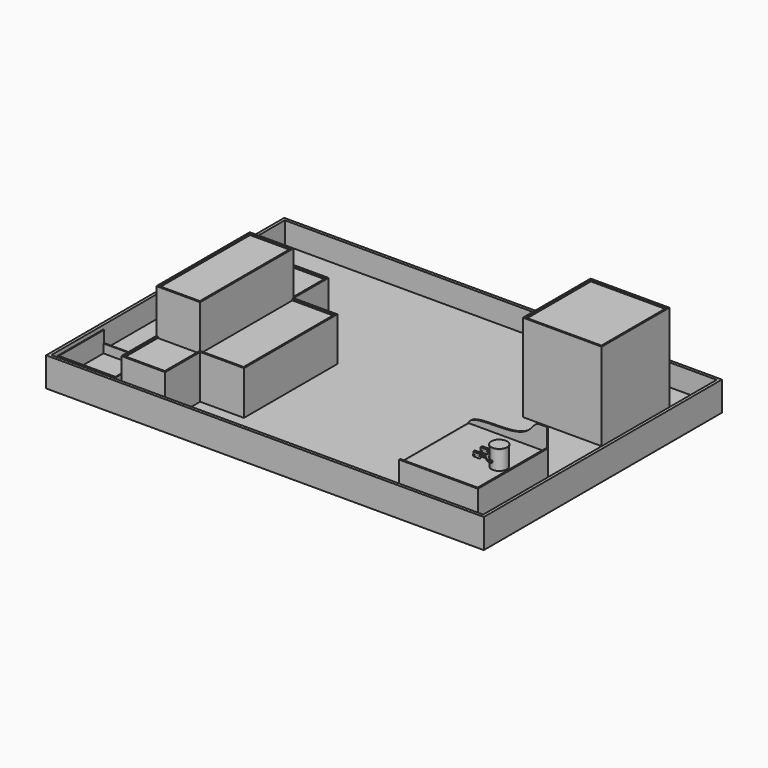
from build123d import *

# Parameters (mm, degrees)
F0_R       = 27.2
F1_DEPTH   = 2.83
F2_R       = 26.4
F3_DEPTH   = 67.36
F4_R       = 27.2
F5_DEPTH   = 2.83
F9_W       = 270
F9_H       = 300
F10_DEPTH  = 72
F12_DEPTH  = 15
F14_DEPTH  = 5
F15_W      = 5
F15_H      = 290
F16_DEPTH  = 5
F17_W      = 1500
F17_H      = 1020
F18_DEPTH  = 25
F19_W      = 270
F19_H      = 290
F20_DEPTH  = 300
F21_W      = 260
F21_H      = 280
F22_DEPTH  = 5
F23_W      = 1500
F23_H      = 1020
F23_W_2    = 1480
F23_H_2    = 1000
F24_DEPTH  = 75
F26_DEPTH  = 150
F27_W      = 150
F27_H      = 400
F28_DEPTH  = 150
F29_W      = 140
F29_H      = 390
F30_DEPTH  = 5
F31_W      = 140
F31_H      = 145
F31_W_2    = 145
F31_H_2    = 390
F32_DEPTH  = 5
F33_R      = 3
F34_DEPTH  = 4
F35_R      = 3.99999
F35_2_R    = 3.99999
F36_R      = 3
F37_DEPTH  = 8
F38_R      = 3
F39_DEPTH  = 8
F40_R      = 3
F40_R_2    = 2.5
F41_DEPTH  = 3
F42_R      = 3
F42_R_2    = 2.5
F43_DEPTH  = 3
F45_DEPTH  = 270.001
F46_W      = 200
F46_H      = 200
F46_W_2    = 194
F46_H_2    = 191
F47_DEPTH  = 30
F49_DEPTH  = 40
F50_R      = 3.0302739223
F50_R_2    = 2.9857883715
F50_R_3    = 3.0752405993
F50_R_4    = 2.9957966751
F10_FACE_W = 260
F10_FACE_H = 290
F51_DEPTH  = 6


# Not quite as in the source:
# - a fillet or chamfer is up to 0.001 mm smaller than in the source, because OpenCascade refuses the exact size
# - a feature names something its author has since deleted; it is built from what else it names


with BuildPart() as f1:
    # F0 (on Top) → F1 (new body)
    with BuildSketch(Plane.XY):
        Circle(F0_R)
    extrude(amount=F1_DEPTH)

    # F2 (on face) → F3 (join)
    with BuildSketch(Plane.XY.offset(2.83)):
        Circle(F2_R)
    extrude(amount=F3_DEPTH)

    # F4 (on face) → F5 (join)
    with BuildSketch(Plane.XY.offset(70.19)):
        Circle(F4_R)
    extrude(amount=F5_DEPTH)


with BuildPart() as f10:
    # F9 (on Top) → F10 (new body)
    with BuildSketch(Plane.XY):
        with Locations((-87.8, 0)):
            Rectangle(F9_W, F9_H)
    extrude(amount=-F10_DEPTH)

    # F11 (on face) → F12 (join)
    with BuildSketch(Plane.XY):
        Polygon((-222.8, -145), (-222.8, -150), (47.2, -150), (47.2, 150), (42.2, 150), (42.2, -145), align=None)
    extrude(amount=F12_DEPTH)

    # F13 (on face) → F14 (join)
    with BuildSketch(Plane(origin=(0, 150, 0), x_dir=(-1, 0, 0), z_dir=(0, 1, 0))):
        with BuildLine():
            Line((-21.3134280931, 81.3575685024), (-47.2, 81.3575685024))
            Line((-47.2, 81.3575685024), (-47.2, -72))
            Line((-47.2, -72), (222.8, -72))
            Line((222.8, -72), (222.8, 0))
            add(Edge.make_bspline(
                [(-21.3134280931, 81.3575685024), (-6.3059147253, 81.3822787863), (12.9585432644, 38.1268753575), (103.6097013063, 23.6068887567), (223.0224295336, 30.7718731823), (222.8, 0)],
                knots=[0, 0, 0, 0, 0.2487100673, 0.6151112321, 1, 1, 1, 1], degree=3))
        make_face()
    extrude(amount=-F14_DEPTH)

    # F15 (on face) → F16 (join)
    with BuildSketch(Plane.XY):
        with Locations((-220.3, 0)):
            Rectangle(F15_W, F15_H)
    extrude(amount=F16_DEPTH)

    # F17 (on face) → F18 (join)
    with BuildSketch(Plane(origin=(0, 0, -72), x_dir=(1, 0, 0), z_dir=(0, 0, -1))):
        with Locations((-602.8, -260)):
            Rectangle(F17_W, F17_H)
    extrude(amount=F18_DEPTH)

    # F19 (on face) → F20 (join)
    with BuildSketch(Plane.XY.offset(-72)):
        with Locations((-87.8, 525)):
            Rectangle(F19_W, F19_H)
    extrude(amount=F20_DEPTH)

    # F21 (on face) → F22 (cut)
    with BuildSketch(Plane.XY.offset(228)):
        with Locations((-87.8, 525)):
            Rectangle(F21_W, F21_H)
    extrude(amount=-F22_DEPTH, mode=Mode.SUBTRACT)

    # F23 (on face) → F24 (join)
    with BuildSketch(Plane.XY.offset(-72)):
        with Locations((-602.8, 260)):
            Rectangle(F23_W, F23_H)
        with Locations((-602.8, 260)):
            Rectangle(F23_W_2, F23_H_2, mode=Mode.SUBTRACT)
    extrude(amount=F24_DEPTH)

    # F25 (on face) → F26 (join)
    with BuildSketch(Plane.XY.offset(-72)):
        Polygon((-952.8, 460), (-1102.8, 460), (-1102.8, -240), (-952.8, -240), (-952.8, -90), (-802.8, -90), (-802.8, 310), (-952.8, 310), align=None)
    extrude(amount=F26_DEPTH)

    # F27 (on face) → F28 (join)
    with BuildSketch(Plane.XY.offset(78)):
        with Locations((-1027.8, 110)):
            Rectangle(F27_W, F27_H)
    extrude(amount=F28_DEPTH)

    # F29 (on face) → F30 (cut)
    with BuildSketch(Plane.XY.offset(228)):
        with Locations((-1027.8, 110)):
            Rectangle(F29_W, F29_H)
    extrude(amount=-F30_DEPTH, mode=Mode.SUBTRACT)

    # F31 (on face) → F32 (cut)
    with BuildSketch(Plane.XY.offset(78)):
        with Locations((-1027.8, 382.5)):
            Rectangle(F31_W, F31_H)
        with Locations((-880.3, 110)):
            Rectangle(F31_W_2, F31_H_2)
        with Locations((-1027.8, -162.5)):
            Rectangle(F31_W, F31_H)
    extrude(amount=-F32_DEPTH, mode=Mode.SUBTRACT)

    # F46 (on face) → F47 (join)
    with BuildSketch(Plane.XY.offset(-72)):
        with Locations((-1232.8, -130)):
            Rectangle(F46_W, F46_H)
        with Locations((-1232.8, -128.5)):
            Rectangle(F46_W_2, F46_H_2, mode=Mode.SUBTRACT)
    extrude(amount=F47_DEPTH)

    # F48 (on face) → F49 (join)
    with BuildSketch(Plane.XY.offset(-42)):
        Polygon((-1329.8, -30), (-1332.8, -30), (-1332.8, -230), (-1329.8, -230), (-1135.8, -230), (-1132.8, -230), (-1132.8, -30), (-1135.8, -30), (-1135.8, -224), (-1329.8, -224), align=None)
    extrude(amount=F49_DEPTH)


with BuildPart() as f34:
    # F33 (on offset) → F34 (new body, symmetric)
    with BuildSketch(Plane.XY.offset(25)):
        with BuildLine():
            Line((-55, -12), (-74.5, -12))
            Line((-74.5, -12), (-74.5, -13))
            Line((-74.5, -13), (-65.6457513111, -13))
            ThreePointArc((-65.6457513111, -13), (-67, -16), (-65.6457513111, -19))
            Line((-65.6457513111, -19), (-74.5, -19))
            Line((-74.5, -19), (-74.5, -20))
            Line((-74.5, -20), (-55, -20))
            ThreePointArc((-55, -20), (-51, -16), (-55, -12))
        make_face()
        with Locations((-63, -16)):
            Circle(F33_R, mode=Mode.SUBTRACT)
        with Locations((-55, -16)):
            Circle(F33_R, mode=Mode.SUBTRACT)
    extrude(amount=F34_DEPTH, both=True)

    # F35 (radius 4 in the source; OpenCascade refuses exactly that, so slightly less here)
    f35_edges = [f34.edges().sort_by_distance(p)[0] for p in [
        (-74.5, -19.5, 29),
        (-74.5, -12.5, 29),
        (-74.5, -19.5, 21),
        (-74.5, -12.5, 21),
    ]]
    fillet(f35_edges, radius=F35_R)

    # F36 (on face) → F37 (join, through all)
    with BuildSketch(Plane.XZ.offset(20)):
        with Locations((-70.5, 25)):
            Circle(F36_R)
    extrude(amount=-F37_DEPTH)

    # F42 (on offset) → F43 (join, symmetric)
    with BuildSketch(Plane.XY.offset(25)):
        with Locations((-63, -16)):
            Circle(F42_R)
        with Locations((-63, -16)):
            Circle(F42_R_2, mode=Mode.SUBTRACT)
        with Locations((-55, -16)):
            Circle(F42_R)
        with Locations((-55, -16)):
            Circle(F42_R_2, mode=Mode.SUBTRACT)
    extrude(amount=F43_DEPTH, both=True)


with BuildPart() as f34b:
    # F33 (on offset) → F34, piece 2 (new body, symmetric)
    with BuildSketch(Plane.XY.offset(25)):
        with BuildLine():
            Line((-74.5, 13), (-74.5, 12))
            Line((-74.5, 12), (-55, 12))
            ThreePointArc((-55, 12), (-51, 16), (-55, 20))
            Line((-55, 20), (-74.5, 20))
            Line((-74.5, 20), (-74.5, 19))
            Line((-74.5, 19), (-65.6457513111, 19))
            ThreePointArc((-65.6457513111, 19), (-67, 16), (-65.6457513111, 13))
            Line((-65.6457513111, 13), (-74.5, 13))
        make_face()
        with Locations((-63, 16)):
            Circle(F33_R, mode=Mode.SUBTRACT)
        with Locations((-55, 16)):
            Circle(F33_R, mode=Mode.SUBTRACT)
    extrude(amount=F34_DEPTH, both=True)

    # F35#2 (radius 4 in the source; OpenCascade refuses exactly that, so slightly less here)
    f35_2_edges = [f34b.edges().sort_by_distance(p)[0] for p in [
        (-74.5, 12.5, 29),
        (-74.5, 19.5, 29),
        (-74.5, 19.5, 21),
        (-74.5, 12.5, 21),
    ]]
    fillet(f35_2_edges, radius=F35_2_R)

    # F38 (on face) → F39 (join, through all)
    with BuildSketch(Plane(origin=(0, 20, 0), x_dir=(-1, 0, 0), z_dir=(0, 1, 0))):
        with Locations((70.5, 25)):
            Circle(F38_R)
    extrude(amount=-F39_DEPTH)

    # F40 (on offset) → F41 (join, symmetric)
    with BuildSketch(Plane.XY.offset(25)):
        with Locations((-55, 16)):
            Circle(F40_R)
        with Locations((-55, 16)):
            Circle(F40_R_2, mode=Mode.SUBTRACT)
        with Locations((-63, 16)):
            Circle(F40_R)
        with Locations((-63, 16)):
            Circle(F40_R_2, mode=Mode.SUBTRACT)
    extrude(amount=F41_DEPTH, both=True)


with BuildPart() as f45_tool:
    # F44 (on face) → F45 (new body, through all)
    with BuildSketch(Plane(origin=(0, 20, 0), x_dir=(-1, 0, 0), z_dir=(0, 1, 0))):
        with BuildLine():
            Line((71.5, 26), (71.5, 27.2912878475))
            ThreePointArc((71.5, 27.2912878475), (70.5, 27.5), (69.5, 27.2912878475))
            Line((69.5, 27.2912878475), (69.5, 26))
            Line((69.5, 26), (68.2087121525, 26))
            ThreePointArc((68.2087121525, 26), (68, 25), (68.2087121525, 24))
            Line((68.2087121525, 24), (69.5, 24))
            Line((69.5, 24), (69.5, 22.7087121525))
            ThreePointArc((69.5, 22.7087121525), (70.5, 22.5), (71.5, 22.7087121525))
            Line((71.5, 22.7087121525), (71.5, 24))
            Line((71.5, 24), (72.7912878475, 24))
            ThreePointArc((72.7912878475, 24), (73, 25), (72.7912878475, 26))
            Line((72.7912878475, 26), (71.5, 26))
        make_face()
    extrude(amount=-F45_DEPTH)


with BuildPart() as f34_1:
    add(f34.part)

    # F45: cut by f45_tool
    add(f45_tool.part, mode=Mode.SUBTRACT)


with BuildPart() as f34b_1:
    add(f34b.part)

    # F45: cut by f45_tool
    add(f45_tool.part, mode=Mode.SUBTRACT)


with BuildPart() as f51:
    # F50 (on face) + F10_face (on face) → F51 (new body)
    with BuildSketch(Plane.XY.offset(29)):
        with BuildLine():
            ThreePointArc((-71.9986608624, 19.9992600828), (-74.119981206, 19.1205804264), (-74.9986608624, 16.9992600828))
            Line((-74.9986608624, 16.9992600828), (-74.9986608624, 14.9319520891))
            ThreePointArc((-74.9986608624, 14.9319520891), (-74.119981206, 12.8106317455), (-71.9986608624, 11.9319520891))
            Line((-71.9986608624, 11.9319520891), (-33.2765181611, 11.9319520891))
            ThreePointArc((-33.2765181611, 11.9319520891), (-35.5474344403, -0.0287606514), (-33.3410842856, -12.0015518465))
            Line((-33.3410842856, -12.0015518465), (-71.5077546412, -12.0054899377))
            ThreePointArc((-71.5077546412, -12.0054899377), (-73.6288748781, -12.8842790214), (-74.507445097, -15.0054899217))
            Line((-74.507445097, -15.0054899217), (-74.507445097, -17.0043950344))
            ThreePointArc((-74.507445097, -17.0043950344), (-73.6286559973, -19.1258248155), (-71.5071355527, -20.0043950184))
            Line((-71.5071355527, -20.0043950184), (-28.9120785892, -20))
            ThreePointArc((-28.9120785892, -20), (-16.5130116876, -30.0834293783), (-0.8348187548, -33.1828929484))
            Line((-0.8348187548, -33.1828929484), (-0.8348187548, -28.1561445445))
            ThreePointArc((-0.8348187548, -28.1561445445), (-28.0066286702, 0.1016434152), (-0.3686239943, 27.9036313295))
            Line((-0.3686239943, 27.9036313295), (-0.3686239943, 32.920781523))
            ThreePointArc((-0.3686239943, 32.920781523), (-16.1670649732, 30.0073032154), (-28.7336144547, 19.9992600828))
            Line((-28.7336144547, 19.9992600828), (-71.9986608624, 19.9992600828))
        make_face()
        with Locations((-63, -16)):
            Circle(F50_R, mode=Mode.SUBTRACT)
        with Locations((-55, -16)):
            Circle(F50_R_2, mode=Mode.SUBTRACT)
        with Locations((-63, 16)):
            Circle(F50_R_3, mode=Mode.SUBTRACT)
        with Locations((-55, 16)):
            Circle(F50_R_4, mode=Mode.SUBTRACT)
    with BuildSketch(Plane(origin=(-87.8, 0, 0), x_dir=(1, 0, 0), z_dir=(0, 0, 1))):
        Rectangle(F10_FACE_W, F10_FACE_H)
    extrude(amount=F51_DEPTH)


solid = Compound([f1.part, f10.part, f34_1.part, f34b_1.part, f51.part])
